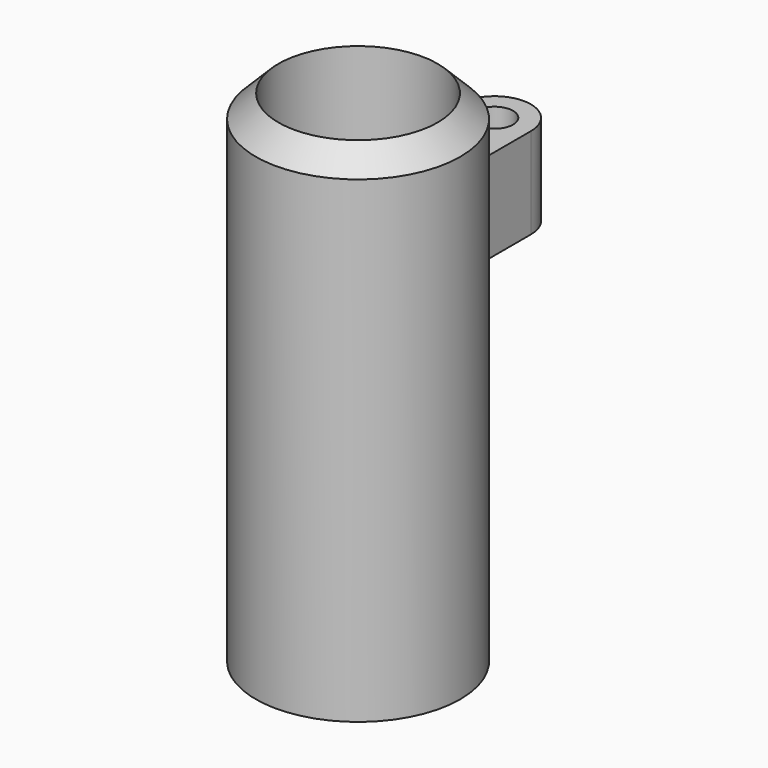
from build123d import *

# Parameters (mm, degrees)
F0_R         = 28.575
F1_DEPTH     = 139.7
F2_T         = -6.35
F5_DEPTH     = 25.4
F7_SIZE      = 6.34999
F8_T4_ANGLE  = 86.6853703019
F8_T11_ANGLE = 86.6853703019


# Not quite as in the source:
# - a fillet or chamfer that OpenCascade refuses, or shapes differently, is made with other operations: its cross-section is extruded or revolved along the edge and cut away or added
# - two fillets or chamfers of one size are made in one step
# - a fillet or chamfer is up to 0.001 mm smaller than in the source, because OpenCascade refuses the exact size


with BuildPart() as f1:
    # F0 (on Top) → F1 (new body)
    with BuildSketch(Plane.XY):
        Circle(F0_R)
    extrude(amount=F1_DEPTH)

    # F2
    f2_openings = [f1.faces().sort_by_distance(p)[0] for p in [
        (0, 0, 139.7),
    ]]
    offset(amount=F2_T, openings=f2_openings)

    # F4 (on offset) → F5 (join)
    with BuildSketch(Plane.XY.offset(114.3)):
        with BuildLine():
            ThreePointArc((10.16, 47.625), (0, 57.785), (-10.16, 47.625))
            ThreePointArc((-10.16, 47.625), (0, 37.465), (10.16, 47.625))
        make_face()
        with BuildLine():
            ThreePointArc((-5.207, 47.625), (0, 52.832), (5.207, 47.625))
            ThreePointArc((5.207, 47.625), (0, 42.418), (-5.207, 47.625))
        make_face(mode=Mode.SUBTRACT)
        with BuildLine():
            ThreePointArc((10.16, 47.625), (0, 37.465), (-10.16, 47.625))
            Line((-10.16, 47.625), (-10.16, 27.305))
            Line((-10.16, 27.305), (10.16, 27.305))
            Line((10.16, 27.305), (10.16, 47.625))
        make_face()
    extrude(amount=-F5_DEPTH)

    # F6: union 

    # F7 (size 6.35 in the source; OpenCascade refuses exactly that, so slightly less here)
    f7_edges = [f1.edges().sort_by_distance(p)[0] for p in [
        (-28.575, 0, 139.7),
    ]]
    chamfer(f7_edges, length=F7_SIZE)

    # F8: chamfer of 5.08 on 3 edges, made by hand


with BuildPart() as f8_tool2:
    # F8_s3 → F8_t4 (revolve)
    with BuildSketch(Plane(origin=(0, 0, 0), x_dir=(0, 0, 1), z_dir=(-0.7272616235, -0.6863603507, 0))):
        Polygon((119.38, 28.575), (114.3, 33.655), (114.3, 28.575), align=None)
    revolve(axis=Axis((0, 0, 114.3), (0, 0, -1)), revolution_arc=F8_T4_ANGLE)

    split(bisect_by=Plane.XZ.offset(-27.305), keep=Keep.BOTTOM)

    split(bisect_by=Plane.YZ.offset(10.16), keep=Keep.BOTTOM)

    split(bisect_by=Plane.YZ.offset(-10.16), keep=Keep.TOP)


with BuildPart() as f1_1:
    add(f1.part)

    # F8_t1: union F8_tool2
    add(f8_tool2.part)


with BuildPart() as f8_tool9:
    # F8_s10 → F8_t11 (revolve)
    with BuildSketch(Plane(origin=(0, 0, 0), x_dir=(0, 0, 1), z_dir=(-0.7272616235, -0.6863603507, 0))):
        Polygon((83.82, 28.575), (88.9, 33.655), (88.9, 28.575), align=None)
    revolve(axis=Axis((0, 0, 88.9), (0, 0, -1)), revolution_arc=F8_T11_ANGLE)

    split(bisect_by=Plane.XZ.offset(-27.305), keep=Keep.BOTTOM)

    split(bisect_by=Plane.YZ.offset(10.16), keep=Keep.BOTTOM)

    split(bisect_by=Plane.YZ.offset(-10.16), keep=Keep.TOP)


with BuildPart() as f1_2:
    add(f1_1.part)

    # F8_t8: union F8_tool9
    add(f8_tool9.part)

    # F8_s15 → F8_t16 (revolve)
    with BuildSketch(Plane.XZ):
        Polygon((22.225, 11.43), (17.145, 6.35), (22.225, 6.35), align=None)
    revolve(axis=Axis((0, 0, 6.35), (0, 0, -1)))


solid = f1_2.part
